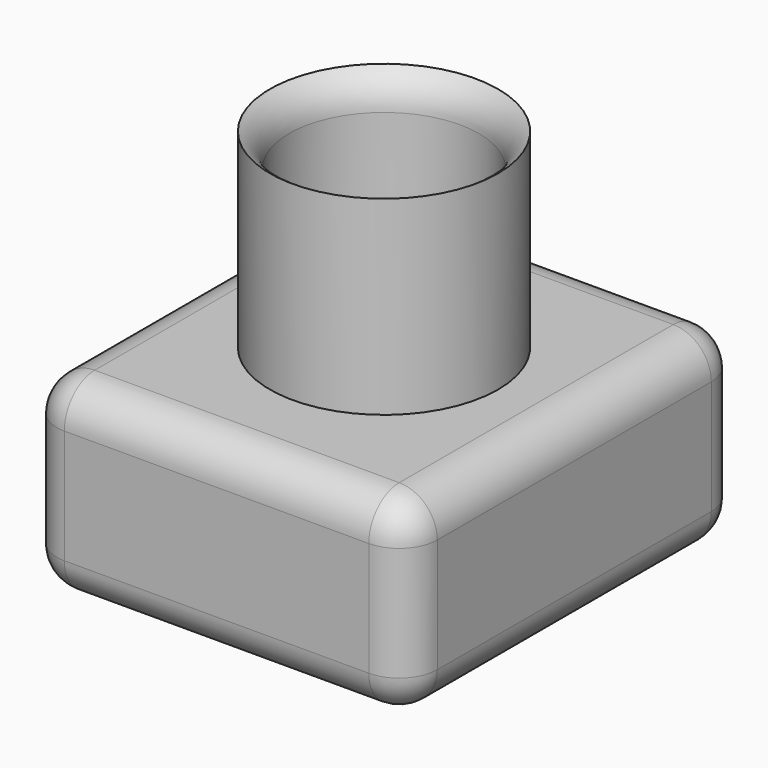
from build123d import *

# Parameters (mm, degrees)
F0_W         = 50
F0_H         = 55
F0_R         = 15
F0_R_2       = 12.5
F1_DEPTH     = 25
F2_DEPTH     = 50
F3_T1_DEPTH  = 40
F3_T3_DEPTH  = 45
F3_T5_DEPTH  = 15
F3_S9_W      = 5.1
F3_S9_H      = 5.1
F3_T10_DEPTH = 5.1
F3_S15_W     = 5.1
F3_S15_H     = 5.1
F3_T16_DEPTH = 5.1
F3_S21_W     = 5.1
F3_S21_H     = 5.1
F3_T22_DEPTH = 5.1
F3_S27_W     = 5.1
F3_S27_H     = 5.1
F3_T28_DEPTH = 5.1
F3_S33_W     = 5.1
F3_S33_H     = 5.1
F3_T34_DEPTH = 5.1
F3_S39_W     = 5.1
F3_S39_H     = 5.1
F3_T40_DEPTH = 5.1
F3_S45_W     = 5.1
F3_S45_H     = 5.1
F3_T46_DEPTH = 5.1
F3_S51_W     = 5.1
F3_S51_H     = 5.1
F3_T52_DEPTH = 5.1


# Not quite as in the source:
# - a fillet or chamfer that OpenCascade refuses, or shapes differently, is made with other operations: its cross-section is extruded or revolved along the edge and cut away or added


with BuildPart() as f1:
    # F0 (on Top) → F1 (new body)
    with BuildSketch(Plane.XY):
        with Locations((-25, 27.5)):
            Rectangle(F0_W, F0_H)
        with Locations((-25, 27.5)):
            Circle(F0_R, mode=Mode.SUBTRACT)
        with Locations((-25, 27.5)):
            Circle(F0_R)
        with Locations((-25, 27.5)):
            Circle(F0_R_2, mode=Mode.SUBTRACT)
        with Locations((-25, 27.5)):
            Circle(F0_R_2)
    extrude(amount=F1_DEPTH)

    # F0 (on Top) → F2 (join)
    with BuildSketch(Plane.XY):
        with Locations((-25, 27.5)):
            Circle(F0_R)
        with Locations((-25, 27.5)):
            Circle(F0_R_2, mode=Mode.SUBTRACT)
    extrude(amount=F2_DEPTH)

    # F3: fillet of radius 5 on 13 edges, made by hand

    # F3_s2 → F3_t1 (cut)
    with BuildSketch(Plane.YZ.offset(-45)):
        with BuildLine():
            ThreePointArc((55, 20), (53.5355339059, 23.5355339059), (50, 25))
            Line((50, 25), (55, 25))
            Line((55, 25), (55, 20))
        make_face()
        with BuildLine():
            ThreePointArc((5, 0), (1.4644660941, 1.4644660941), (0, 5))
            Line((0, 5), (0, 0))
            Line((0, 0), (5, 0))
        make_face()
        with BuildLine():
            ThreePointArc((5, 25), (1.4644660941, 23.5355339059), (0, 20))
            Line((0, 20), (0, 25))
            Line((0, 25), (5, 25))
        make_face()
        with BuildLine():
            ThreePointArc((55, 5), (53.5355339059, 1.4644660941), (50, 0))
            Line((50, 0), (55, 0))
            Line((55, 0), (55, 5))
        make_face()
    extrude(amount=F3_T1_DEPTH, mode=Mode.SUBTRACT)

    # F3_s4 → F3_t3 (cut)
    with BuildSketch(Plane.XZ.offset(-50)):
        with BuildLine():
            ThreePointArc((-50, 20), (-48.5355339059, 23.5355339059), (-45, 25))
            Line((-45, 25), (-50, 25))
            Line((-50, 25), (-50, 20))
        make_face()
        with BuildLine():
            ThreePointArc((0, 5), (-1.4644660941, 1.4644660941), (-5, 0))
            Line((-5, 0), (0, 0))
            Line((0, 0), (0, 5))
        make_face()
        with BuildLine():
            ThreePointArc((0, 20), (-1.4644660941, 23.5355339059), (-5, 25))
            Line((-5, 25), (0, 25))
            Line((0, 25), (0, 20))
        make_face()
        with BuildLine():
            ThreePointArc((-50, 5), (-48.5355339059, 1.4644660941), (-45, 0))
            Line((-45, 0), (-50, 0))
            Line((-50, 0), (-50, 5))
        make_face()
    extrude(amount=F3_T3_DEPTH, mode=Mode.SUBTRACT)

    # F3_s6 → F3_t5 (cut)
    with BuildSketch(Plane.XY.offset(5)):
        with BuildLine():
            ThreePointArc((-50, 5), (-48.5355339059, 1.4644660941), (-45, 0))
            Line((-45, 0), (-50, 0))
            Line((-50, 0), (-50, 5))
        make_face()
        with BuildLine():
            ThreePointArc((0, 5), (-1.4644660941, 1.4644660941), (-5, 0))
            Line((-5, 0), (0, 0))
            Line((0, 0), (0, 5))
        make_face()
        with BuildLine():
            ThreePointArc((-5, 55), (-1.4644660941, 53.5355339059), (0, 50))
            Line((0, 50), (0, 55))
            Line((0, 55), (-5, 55))
        make_face()
        with BuildLine():
            ThreePointArc((-45, 55), (-48.5355339059, 53.5355339059), (-50, 50))
            Line((-50, 50), (-50, 55))
            Line((-50, 55), (-45, 55))
        make_face()
    extrude(amount=F3_T5_DEPTH, mode=Mode.SUBTRACT)


with BuildPart() as f3_tool8:
    # F3_s9 → F3_t10 (new body)
    with BuildSketch(Plane.XZ.offset(-50)):
        with Locations((-2.45, 22.55)):
            Rectangle(F3_S9_W, F3_S9_H)
    extrude(amount=-F3_T10_DEPTH)

    # F3_s11 → F3_t12 (revolve, cut)
    with BuildSketch(Plane(origin=(-5, 50, 20), x_dir=(-0.7071067812, 0, -0.7071067812), z_dir=(0.7071067812, 0, -0.7071067812))):
        with BuildLine():
            ThreePointArc((0, -5), (5, 0), (0, 5))
            Line((0, 5), (0, -5))
        make_face()
    revolve(axis=Axis((-5, 50, 20), (0, 1, 0)), mode=Mode.SUBTRACT)


with BuildPart() as f1_1:
    add(f1.part)

    # F3_t7: cut F3_tool8
    add(f3_tool8.part, mode=Mode.SUBTRACT)


with BuildPart() as f3_tool14:
    # F3_s15 → F3_t16 (new body)
    with BuildSketch(Plane.XZ.offset(-50)):
        with Locations((-47.55, 22.55)):
            Rectangle(F3_S15_W, F3_S15_H)
    extrude(amount=-F3_T16_DEPTH)

    # F3_s17 → F3_t18 (revolve, cut)
    with BuildSketch(Plane(origin=(-45, 50, 20), x_dir=(0.7071067812, 0, -0.7071067812), z_dir=(0.7071067812, 0, 0.7071067812))):
        with BuildLine():
            ThreePointArc((0, -5), (5, 0), (0, 5))
            Line((0, 5), (0, -5))
        make_face()
    revolve(axis=Axis((-45, 50, 20), (0, 1, 0)), mode=Mode.SUBTRACT)


with BuildPart() as f1_2:
    add(f1_1.part)

    # F3_t13: cut F3_tool14
    add(f3_tool14.part, mode=Mode.SUBTRACT)


with BuildPart() as f3_tool20:
    # F3_s21 → F3_t22 (new body)
    with BuildSketch(Plane.YZ.offset(-45)):
        with Locations((2.45, 22.55)):
            Rectangle(F3_S21_W, F3_S21_H)
    extrude(amount=-F3_T22_DEPTH)

    # F3_s23 → F3_t24 (revolve, cut)
    with BuildSketch(Plane(origin=(-45, 5, 20), x_dir=(0, 0.7071067812, -0.7071067812), z_dir=(0, 0.7071067812, 0.7071067812))):
        with BuildLine():
            ThreePointArc((0, -5), (5, 0), (0, 5))
            Line((0, 5), (0, -5))
        make_face()
    revolve(axis=Axis((-45, 5, 20), (-1, 0, 0)), mode=Mode.SUBTRACT)


with BuildPart() as f1_3:
    add(f1_2.part)

    # F3_t19: cut F3_tool20
    add(f3_tool20.part, mode=Mode.SUBTRACT)


with BuildPart() as f3_tool26:
    # F3_s27 → F3_t28 (new body)
    with BuildSketch(Plane.YZ.offset(-45)):
        with Locations((2.45, 2.45)):
            Rectangle(F3_S27_W, F3_S27_H)
    extrude(amount=-F3_T28_DEPTH)

    # F3_s29 → F3_t30 (revolve, cut)
    with BuildSketch(Plane(origin=(-45, 5, 5), x_dir=(0, 0.7071067812, 0.7071067812), z_dir=(0, -0.7071067812, 0.7071067812))):
        with BuildLine():
            ThreePointArc((0, -5), (5, 0), (0, 5))
            Line((0, 5), (0, -5))
        make_face()
    revolve(axis=Axis((-45, 5, 5), (-1, 0, 0)), mode=Mode.SUBTRACT)


with BuildPart() as f1_4:
    add(f1_3.part)

    # F3_t25: cut F3_tool26
    add(f3_tool26.part, mode=Mode.SUBTRACT)


with BuildPart() as f3_tool32:
    # F3_s33 → F3_t34 (new body)
    with BuildSketch(Plane.YZ.offset(-5)):
        with Locations((2.45, 2.45)):
            Rectangle(F3_S33_W, F3_S33_H)
    extrude(amount=F3_T34_DEPTH)

    # F3_s35 → F3_t36 (revolve, cut)
    with BuildSketch(Plane(origin=(-5, 5, 5), x_dir=(0, 0.7071067812, 0.7071067812), z_dir=(0, 0.7071067812, -0.7071067812))):
        with BuildLine():
            ThreePointArc((0, -5), (5, 0), (0, 5))
            Line((0, 5), (0, -5))
        make_face()
    revolve(axis=Axis((-5, 5, 5), (1, 0, 0)), mode=Mode.SUBTRACT)


with BuildPart() as f1_5:
    add(f1_4.part)

    # F3_t31: cut F3_tool32
    add(f3_tool32.part, mode=Mode.SUBTRACT)


with BuildPart() as f3_tool38:
    # F3_s39 → F3_t40 (new body)
    with BuildSketch(Plane.YZ.offset(-5)):
        with Locations((2.45, 22.55)):
            Rectangle(F3_S39_W, F3_S39_H)
    extrude(amount=F3_T40_DEPTH)

    # F3_s41 → F3_t42 (revolve, cut)
    with BuildSketch(Plane(origin=(-5, 5, 20), x_dir=(0, 0.7071067812, -0.7071067812), z_dir=(0, -0.7071067812, -0.7071067812))):
        with BuildLine():
            ThreePointArc((0, -5), (5, 0), (0, 5))
            Line((0, 5), (0, -5))
        make_face()
    revolve(axis=Axis((-5, 5, 20), (1, 0, 0)), mode=Mode.SUBTRACT)


with BuildPart() as f1_6:
    add(f1_5.part)

    # F3_t37: cut F3_tool38
    add(f3_tool38.part, mode=Mode.SUBTRACT)


with BuildPart() as f3_tool44:
    # F3_s45 → F3_t46 (new body)
    with BuildSketch(Plane.XZ.offset(-50)):
        with Locations((-2.45, 2.45)):
            Rectangle(F3_S45_W, F3_S45_H)
    extrude(amount=-F3_T46_DEPTH)

    # F3_s47 → F3_t48 (revolve, cut)
    with BuildSketch(Plane(origin=(-5, 50, 5), x_dir=(-0.7071067812, 0, 0.7071067812), z_dir=(-0.7071067812, 0, -0.7071067812))):
        with BuildLine():
            ThreePointArc((0, -5), (5, 0), (0, 5))
            Line((0, 5), (0, -5))
        make_face()
    revolve(axis=Axis((-5, 50, 5), (0, 1, 0)), mode=Mode.SUBTRACT)


with BuildPart() as f1_7:
    add(f1_6.part)

    # F3_t43: cut F3_tool44
    add(f3_tool44.part, mode=Mode.SUBTRACT)


with BuildPart() as f3_tool50:
    # F3_s51 → F3_t52 (new body)
    with BuildSketch(Plane.XZ.offset(-50)):
        with Locations((-47.55, 2.45)):
            Rectangle(F3_S51_W, F3_S51_H)
    extrude(amount=-F3_T52_DEPTH)

    # F3_s53 → F3_t54 (revolve, cut)
    with BuildSketch(Plane(origin=(-45, 50, 5), x_dir=(0.7071067812, 0, 0.7071067812), z_dir=(-0.7071067812, 0, 0.7071067812))):
        with BuildLine():
            ThreePointArc((0, -5), (5, 0), (0, 5))
            Line((0, 5), (0, -5))
        make_face()
    revolve(axis=Axis((-45, 50, 5), (0, 1, 0)), mode=Mode.SUBTRACT)


with BuildPart() as f1_8:
    add(f1_7.part)

    # F3_t49: cut F3_tool50
    add(f3_tool50.part, mode=Mode.SUBTRACT)

    # F3_s55 → F3_t56 (revolve, cut)
    with BuildSketch(Plane.XZ.offset(-27.5)):
        with BuildLine():
            ThreePointArc((-10, 50), (-11.8301270189, 48.1698729811), (-12.5, 45.6698729811))
            Line((-12.5, 45.6698729811), (-12.5, 50))
            Line((-12.5, 50), (-10, 50))
        make_face()
    revolve(axis=Axis((-25, 27.5, 50), (0, 0, 1)), mode=Mode.SUBTRACT)


solid = f1_8.part
